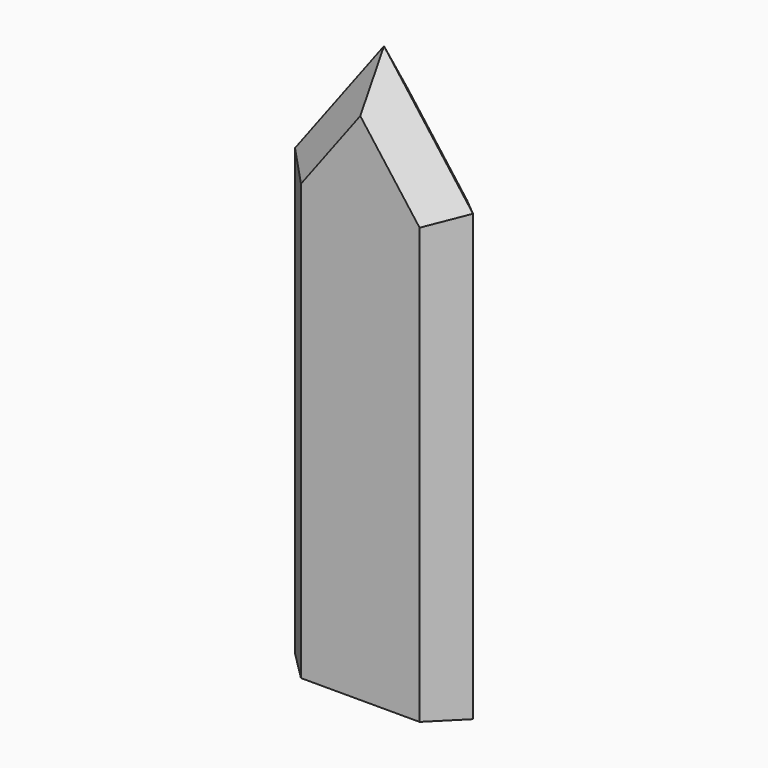
from build123d import *

# Parameters (mm, degrees)
F1_DEPTH = 10
F2_SIZE  = 4.99999
F4_D     = 5
F4_DEPTH = 20
F4_TIP   = 1.5021515476


# Not quite as in the source:
# - a fillet or chamfer is up to 0.001 mm smaller than in the source, because OpenCascade refuses the exact size


with BuildPart() as f1:
    # F0 (on Front) → F1 (new body)
    with BuildSketch(Plane.XZ):
        Polygon((0, 60.1269584066), (-15, 40.1269584066), (-15, -34.8730415934), (15, -34.8730415934), (15, 40.1269584066), align=None)
    extrude(amount=F1_DEPTH)

    # F2 (size 5 in the source; OpenCascade refuses exactly that, so slightly less here)
    f2_edges = [f1.edges().sort_by_distance(p)[0] for p in [
        (-15, -10, 2.626958),
        (-15, 0, 2.626958),
        (-7.5, -10, 50.126958),
        (-7.5, 0, 50.126958),
        (7.5, -10, 50.126958),
        (7.5, 0, 50.126958),
        (15, -10, 2.626958),
        (15, 0, 2.626958),
    ]]
    chamfer(f2_edges, length=F2_SIZE)

    # F4
    with Locations(Plane(origin=(0, 0, -34.8730415934), x_dir=(1, 0, 0), z_dir=(0, 0, -1))):
        with Locations((0, 5.1561156288)):
            Hole(F4_D / 2, depth=F4_DEPTH)
            with Locations((0, 0, -(F4_DEPTH + F4_TIP / 2))):  # 118° drill point
                Cone(0, F4_D / 2, F4_TIP, mode=Mode.SUBTRACT)


solid = f1.part
